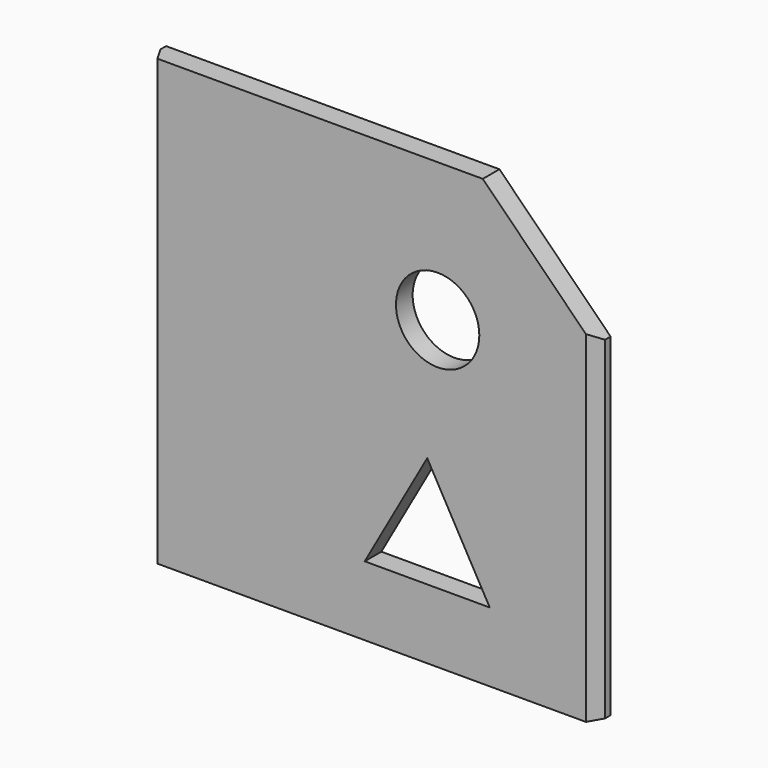
from build123d import *

# Parameters (mm, degrees)
F0_R     = 19.05
F1_DEPTH = 9.525
F2_SIZE2 = 3.6661742094
F2_SIZE  = 6.35
F3_SIZE2 = 3.6661742094
F3_SIZE  = 6.35


# Not quite as in the source:
# - a length typed as a fraction of an inch, garbled in the dataset ("3 / 203.2 mm" for 3/8 in), is restored


with BuildPart() as f1:
    # F0 (on Front) → F1 (new body)
    with BuildSketch(Plane.XZ):
        Polygon((68.2071738782, 117.0869429827), (-84.1928261218, 117.0869429827), (-84.1928261218, -86.1130570173), (119.0071738782, -86.1130570173), (119.0071738782, 66.2869429827), align=None)
        Polygon((14.2321738782, -54.3630570173), (42.8071738782, -3.5630570173), (71.3821738782, -54.3630570173), align=None, mode=Mode.SUBTRACT)
        with Locations((47.5696738782, 53.5869429827)):
            Circle(F0_R, mode=Mode.SUBTRACT)
    extrude(amount=F1_DEPTH)

    # F2
    f2_edges = [f1.edges().sort_by_distance(p)[0] for p in [
        (119.007174, -9.525, -9.913057),
    ]]
    f2_side = f1.faces().sort_by_distance((119.007174, -4.7625, -9.913057))[0]
    chamfer(f2_edges, length=F2_SIZE, length2=F2_SIZE2, reference=f2_side)

    # F3
    f3_edges = [f1.edges().sort_by_distance(p)[0] for p in [
        (-84.192826, -9.525, 15.486943),
    ]]
    f3_side = f1.faces().sort_by_distance((-84.192826, -4.7625, 15.486943))[0]
    chamfer(f3_edges, length=F3_SIZE, length2=F3_SIZE2, reference=f3_side)


solid = f1.part
